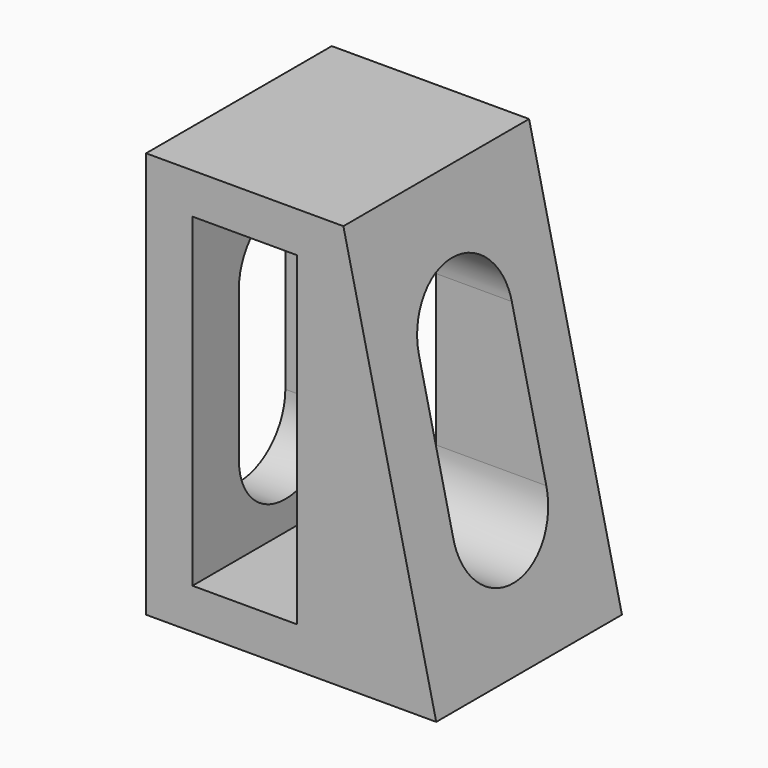
from build123d import *

# Parameters (mm, degrees)
F0_W     = 25
F0_H     = 35
F1_DEPTH = 10
F2_SIZE2 = 34.99999
F2_SIZE  = 7.99999
F3_W     = 9
F3_H     = 28
F4_DEPTH = 33.35697
F5_W     = 10
F5_H     = 13
F6_DEPTH = 25


# Not quite as in the source:
# - a fillet or chamfer is up to 0.001 mm smaller than in the source, because OpenCascade refuses the exact size


with BuildPart() as f1:
    # F0 (on Front) → F1 (new body, symmetric)
    with BuildSketch(Plane.XZ):
        with Locations((-14.1274514172, 17.5)):
            Rectangle(F0_W, F0_H)
    extrude(amount=F1_DEPTH, both=True)

    # F2 (size 8 and 35 in the source; OpenCascade refuses exactly that, so slightly less here)
    f2_edges = [f1.edges().sort_by_distance(p)[0] for p in [
        (-1.627451, 0, 35),
    ]]
    f2_side = f1.faces().sort_by_distance((-14.127451, 0, 35))[0]
    chamfer(f2_edges, length=F2_SIZE, length2=F2_SIZE2, reference=f2_side)

    # F3 (on face) → F4 (cut)
    with BuildSketch(Plane(origin=(0, 10, 0), x_dir=(-1, 0, 0), z_dir=(0, 1, 0))):
        with Locations((18.1274514172, 17.5)):
            Rectangle(F3_W, F3_H)
    extrude(amount=-F4_DEPTH, mode=Mode.SUBTRACT)

    # F5 (on face) → F6 (cut)
    with BuildSketch(Plane(origin=(-26.6274514172, 0, 0), x_dir=(0, -1, 0), z_dir=(-1, 0, 0))):
        with BuildLine():
            ThreePointArc((5, 24), (0, 29), (-5, 24))
            Line((-5, 24), (5, 24))
        make_face()
        with Locations((0, 17.5)):
            Rectangle(F5_W, F5_H)
        with BuildLine():
            Line((5, 11), (-5, 11))
            ThreePointArc((-5, 11), (0, 6), (5, 11))
        make_face()
    extrude(amount=-F6_DEPTH, mode=Mode.SUBTRACT)


solid = f1.part
